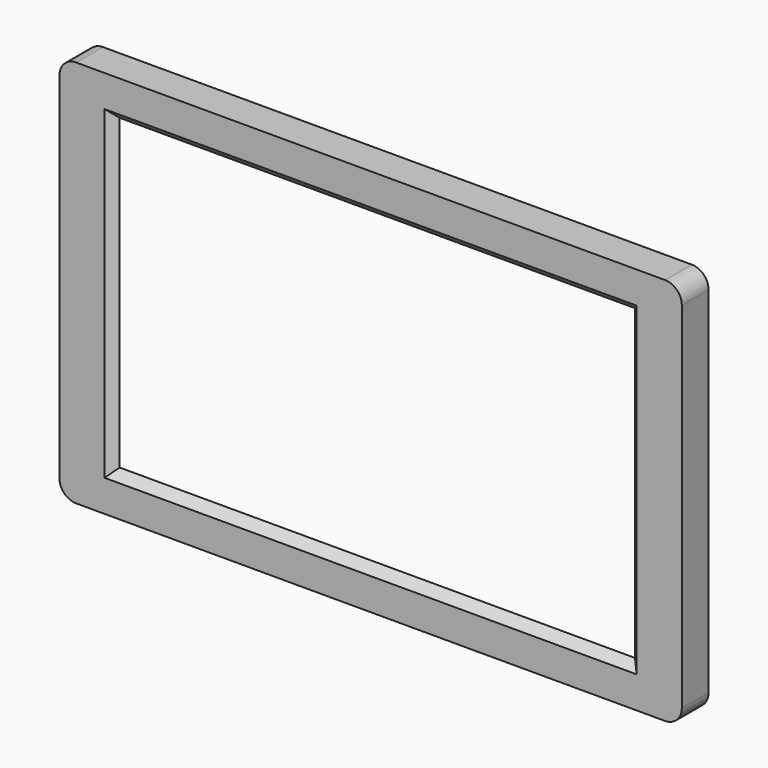
from build123d import *

# Parameters (mm, degrees)
F0_W     = 186
F0_H     = 116
F0_W_2   = 166
F0_H_2   = 106
F1_DEPTH = 10
F0_W_3   = 164
F0_H_3   = 102
F2_DEPTH = 2.5
F0_W_4   = 154
F0_H_4   = 92
F3_DEPTH = 2.5
F4_SIZE  = 2.49999
F5_R     = 5


# Not quite as in the source:
# - a fillet or chamfer is up to 0.001 mm smaller than in the source, because OpenCascade refuses the exact size


with BuildPart() as f1:
    # F0 (on Front) → F1 (new body)
    with BuildSketch(Plane.XZ):
        Rectangle(F0_W, F0_H)
        Rectangle(F0_W_2, F0_H_2, mode=Mode.SUBTRACT)
    extrude(amount=-F1_DEPTH)

    # F0 (on Front) → F2 (join)
    with BuildSketch(Plane.XZ):
        Rectangle(F0_W_2, F0_H_2)
        Rectangle(F0_W_3, F0_H_3, mode=Mode.SUBTRACT)
    extrude(amount=-F2_DEPTH)

    # F0 (on Front) → F3 (join)
    with BuildSketch(Plane.XZ):
        Rectangle(F0_W_3, F0_H_3)
        Rectangle(F0_W_4, F0_H_4, mode=Mode.SUBTRACT)
    extrude(amount=-F3_DEPTH)

    # F4 (size 2.5 in the source; OpenCascade refuses exactly that, so slightly less here)
    f4_edges = [f1.edges().sort_by_distance(p)[0] for p in [
        (0, 0, 46),
        (-77, 0, 0),
        (0, 0, -46),
        (77, 0, 0),
    ]]
    chamfer(f4_edges, length=F4_SIZE)

    # F5
    f5_edges = [f1.edges().sort_by_distance(p)[0] for p in [
        (-93, 5, 58),
        (-93, 5, -58),
        (93, 5, -58),
        (93, 5, 58),
    ]]
    fillet(f5_edges, radius=F5_R)


solid = f1.part
